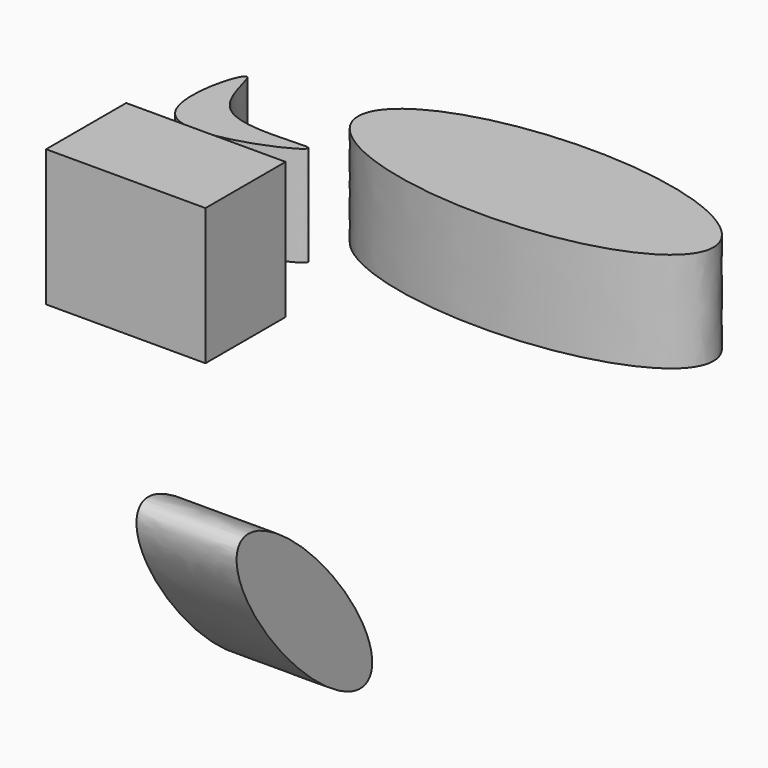
from build123d import *

# Parameters (mm, degrees)
F0_W     = 40.4382697307
F0_H     = 34.6613712609
F1_DEPTH = 25.4
F3_DEPTH = 25.4
F5_DEPTH = 25.4
F7_DEPTH = 25.4


with BuildPart() as f1:
    # F0 (on Front) → F1 (new body)
    with BuildSketch(Plane.XZ):
        with Locations((-28.0179430265, 22.3854687065)):
            Rectangle(F0_W, F0_H)
    extrude(amount=F1_DEPTH)


with BuildPart() as f3:
    # F2 (on Right) → F3 (new body)
    with BuildSketch(Plane.YZ):
        with BuildLine():
            add(Edge.make_bspline(
                [(-55.7470396161, -11.6982134059), (-68.3714359002, -22.4751358886), (-31.7305393019, -52.6145824248), (4.9103572965, -82.7540289611), (-19.1061430178, -41.8376599421), (-43.122643332, -0.9212909232), (-55.7470396161, -11.6982134059)],
                knots=[0, 0, 0, 2.0943951024, 2.0943951024, 4.1887902048, 4.1887902048, 6.2831853072, 6.2831853072, 6.2831853072], degree=2, weights=[1, 0.5, 1, 0.5, 1, 0.5, 1]))
        make_face()
    extrude(amount=F3_DEPTH)


with BuildPart() as f5:
    # F4 (on Top) → F5 (new body)
    with BuildSketch(Plane.XY):
        with BuildLine():
            add(Edge.make_bspline(
                [(-25.996029377, 45.7818955183), (-25.996029377, 15.2350073678), (41.5936456993, 30.508451443), (109.1833207756, 45.7818955183), (41.5936456993, 61.0553395936), (-25.996029377, 76.3287836688), (-25.996029377, 45.7818955183)],
                knots=[0, 0, 0, 2.0943951024, 2.0943951024, 4.1887902048, 4.1887902048, 6.2831853072, 6.2831853072, 6.2831853072], degree=2, weights=[1, 0.5, 1, 0.5, 1, 0.5, 1]))
        make_face()
    extrude(amount=F5_DEPTH)


with BuildPart() as f7:
    # F6 (on Top) → F7 (new body)
    with BuildSketch(Plane.XY):
        with BuildLine():
            add(Edge.make_bspline(
                [(-54.0139712393, 45.2042035758), (-55.9220366105, 44.4010836619), (-65.2943540455, 9.0054192386), (-7.193281723, 34.8499323766), (-52.66189627, 23.6112015522), (-52.4274428558, 45.8719860105), (-54.0139712393, 45.2042035758)],
                knots=[0, 0, 0, 0, 0.2516606354, 0.5412804564, 0.7907478711, 1, 1, 1, 1], degree=3))
        make_face()
    extrude(amount=F7_DEPTH)


solid = Compound([f1.part, f3.part, f5.part, f7.part])
